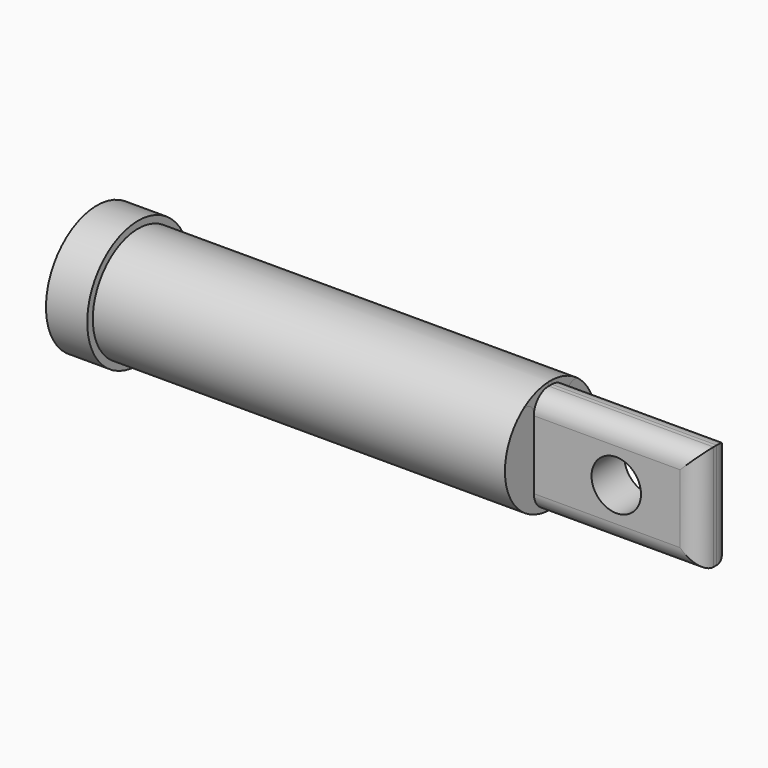
from build123d import *

# Parameters (mm, degrees)
F0_R     = 3.9243
F1_DEPTH = 2.54
F2_R     = 3.4925
F3_DEPTH = 25.4
F4_W     = 2.531840682
F4_H     = 6.5099929156
F5_DEPTH = 10.16
F6_R     = 1.524
F7_DEPTH = 25.4
F8_R     = 1.14299


# Not quite as in the source:
# - a fillet or chamfer is up to 0.001 mm smaller than in the source, because OpenCascade refuses the exact size


with BuildPart() as f1:
    # F0 (on Right) → F1 (new body)
    with BuildSketch(Plane.YZ):
        Circle(F0_R)
    extrude(amount=F1_DEPTH)

    # F2 (on face) → F3 (join)
    with BuildSketch(Plane.YZ.offset(2.54)):
        Circle(F2_R)
    extrude(amount=F3_DEPTH)

    # F4 (on face) → F5 (join)
    with BuildSketch(Plane.YZ.offset(27.94)):
        Rectangle(F4_W, F4_H)
    extrude(amount=F5_DEPTH)

    # F6 (on face) → F7 (cut)
    with BuildSketch(Plane(origin=(0, 1.265920341, 0), x_dir=(-1, 0, 0), z_dir=(0, 1, 0))):
        with Locations((-33.02, 0)):
            Circle(F6_R)
    extrude(amount=-F7_DEPTH, mode=Mode.SUBTRACT)

    # F8 (radius 1.143 in the source; OpenCascade refuses exactly that, so slightly less here)
    f8_edges = [f1.edges().sort_by_distance(p)[0] for p in [
        (38.1, 1.26592, 0),
        (38.1, -1.26592, 0),
        (33.02, 1.26592, 3.254996),
        (33.02, -1.26592, 3.254996),
        (33.02, 1.26592, -3.254996),
        (33.02, -1.26592, -3.254996),
    ]]
    fillet(f8_edges, radius=F8_R)


solid = f1.part
